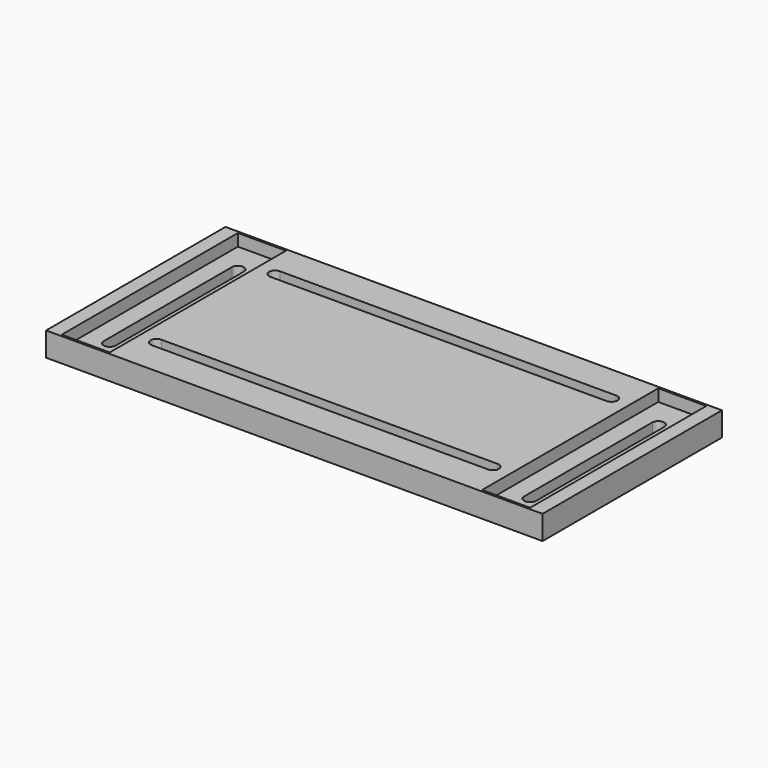
from build123d import *

# Parameters (mm, degrees)
F0_W     = 196.85
F0_H     = 88.9
F1_DEPTH = 9.525
F3_DEPTH = 25.4
F4_W     = 19.05
F4_H     = 87.3125
F5_DEPTH = 4.7625


# Not quite as in the source:
# - a length typed as a fraction of an inch, garbled in the dataset ("3 / 203.2 mm" for 3/8 in), is restored


with BuildPart() as f1:
    # F0 (on Top) → F1 (new body)
    with BuildSketch(Plane.XY):
        with Locations((98.425, 44.45)):
            Rectangle(F0_W, F0_H)
    extrude(amount=F1_DEPTH)

    # F2 (on face) → F3 (cut)
    with BuildSketch(Plane.XY.offset(9.525)):
        with BuildLine():
            ThreePointArc((17.4625, 12.7), (15.08125, 15.08125), (12.7, 12.7))
            Line((12.7, 12.7), (17.4625, 12.7))
        make_face()
        with BuildLine():
            Line((12.7, 76.2), (12.7, 12.7))
            ThreePointArc((12.7, 12.7), (15.08125, 15.08125), (17.4625, 12.7))
            Line((17.4625, 12.7), (17.4625, 76.2))
            ThreePointArc((17.4625, 76.2), (15.08125, 73.81875), (12.7, 76.2))
        make_face()
        with BuildLine():
            Line((17.4625, 12.7), (12.7, 12.7))
            ThreePointArc((12.7, 12.7), (15.08125, 10.31875), (17.4625, 12.7))
        make_face()
        with BuildLine():
            ThreePointArc((17.4625, 76.2), (15.08125, 78.58125), (12.7, 76.2))
            Line((12.7, 76.2), (17.4625, 76.2))
        make_face()
        with BuildLine():
            Line((17.4625, 76.2), (12.7, 76.2))
            ThreePointArc((12.7, 76.2), (15.08125, 73.81875), (17.4625, 76.2))
        make_face()
        with BuildLine():
            ThreePointArc((179.3875, 12.7), (181.76875, 10.31875), (184.15, 12.7))
            Line((184.15, 12.7), (179.3875, 12.7))
        make_face()
        with BuildLine():
            ThreePointArc((179.3875, 12.7), (181.76875, 15.08125), (184.15, 12.7))
            Line((184.15, 12.7), (184.15, 76.2))
            ThreePointArc((184.15, 76.2), (181.76875, 73.81875), (179.3875, 76.2))
            Line((179.3875, 76.2), (179.3875, 12.7))
        make_face()
        with BuildLine():
            Line((179.3875, 12.7), (184.15, 12.7))
            ThreePointArc((184.15, 12.7), (181.76875, 15.08125), (179.3875, 12.7))
        make_face()
        with BuildLine():
            ThreePointArc((179.3875, 76.2), (181.76875, 73.81875), (184.15, 76.2))
            Line((184.15, 76.2), (179.3875, 76.2))
        make_face()
        with BuildLine():
            Line((179.3875, 76.2), (184.15, 76.2))
            ThreePointArc((184.15, 76.2), (181.76875, 78.58125), (179.3875, 76.2))
        make_face()
        with BuildLine():
            ThreePointArc((34.13125, 73.81875), (33.4337980227, 75.5025480227), (31.75, 76.2))
            Line((31.75, 76.2), (31.75, 71.4375))
            ThreePointArc((31.75, 71.4375), (33.4337980227, 72.1349519773), (34.13125, 73.81875))
        make_face()
        with BuildLine():
            Line((165.1, 76.2), (31.75, 76.2))
            ThreePointArc((31.75, 76.2), (33.4337980227, 75.5025480227), (34.13125, 73.81875))
            ThreePointArc((34.13125, 73.81875), (33.4337980227, 72.1349519773), (31.75, 71.4375))
            Line((31.75, 71.4375), (165.1, 71.4375))
            ThreePointArc((165.1, 71.4375), (162.71875, 73.81875), (165.1, 76.2))
        make_face()
        with BuildLine():
            Line((31.75, 71.4375), (31.75, 76.2))
            ThreePointArc((31.75, 76.2), (29.36875, 73.81875), (31.75, 71.4375))
        make_face()
        with BuildLine():
            ThreePointArc((167.48125, 73.81875), (166.7837980227, 75.5025480227), (165.1, 76.2))
            Line((165.1, 76.2), (165.1, 71.4375))
            ThreePointArc((165.1, 71.4375), (166.7837980227, 72.1349519773), (167.48125, 73.81875))
        make_face()
        with BuildLine():
            Line((165.1, 71.4375), (165.1, 76.2))
            ThreePointArc((165.1, 76.2), (162.71875, 73.81875), (165.1, 71.4375))
        make_face()
        with BuildLine():
            ThreePointArc((34.13125, 15.08125), (33.4337980227, 16.7650480227), (31.75, 17.4625))
            Line((31.75, 17.4625), (31.75, 12.7))
            ThreePointArc((31.75, 12.7), (33.4337980227, 13.3974519773), (34.13125, 15.08125))
        make_face()
        with BuildLine():
            Line((165.1, 17.4625), (31.75, 17.4625))
            ThreePointArc((31.75, 17.4625), (33.4337980227, 16.7650480227), (34.13125, 15.08125))
            ThreePointArc((34.13125, 15.08125), (33.4337980227, 13.3974519773), (31.75, 12.7))
            Line((31.75, 12.7), (165.1, 12.7))
            ThreePointArc((165.1, 12.7), (162.71875, 15.08125), (165.1, 17.4625))
        make_face()
        with BuildLine():
            Line((31.75, 12.7), (31.75, 17.4625))
            ThreePointArc((31.75, 17.4625), (29.36875, 15.08125), (31.75, 12.7))
        make_face()
        with BuildLine():
            ThreePointArc((167.48125, 15.08125), (166.7837980227, 16.7650480227), (165.1, 17.4625))
            Line((165.1, 17.4625), (165.1, 12.7))
            ThreePointArc((165.1, 12.7), (166.7837980227, 13.3974519773), (167.48125, 15.08125))
        make_face()
        with BuildLine():
            Line((165.1, 12.7), (165.1, 17.4625))
            ThreePointArc((165.1, 17.4625), (162.71875, 15.08125), (165.1, 12.7))
        make_face()
    extrude(amount=-F3_DEPTH, mode=Mode.SUBTRACT)

    # F4 (on face) → F5 (cut)
    with BuildSketch(Plane.XY.offset(9.525)):
        with Locations((15.08125, 44.45)):
            Rectangle(F4_W, F4_H)
        with Locations((181.76875, 44.45)):
            Rectangle(F4_W, F4_H)
    extrude(amount=-F5_DEPTH, mode=Mode.SUBTRACT)


solid = f1.part
